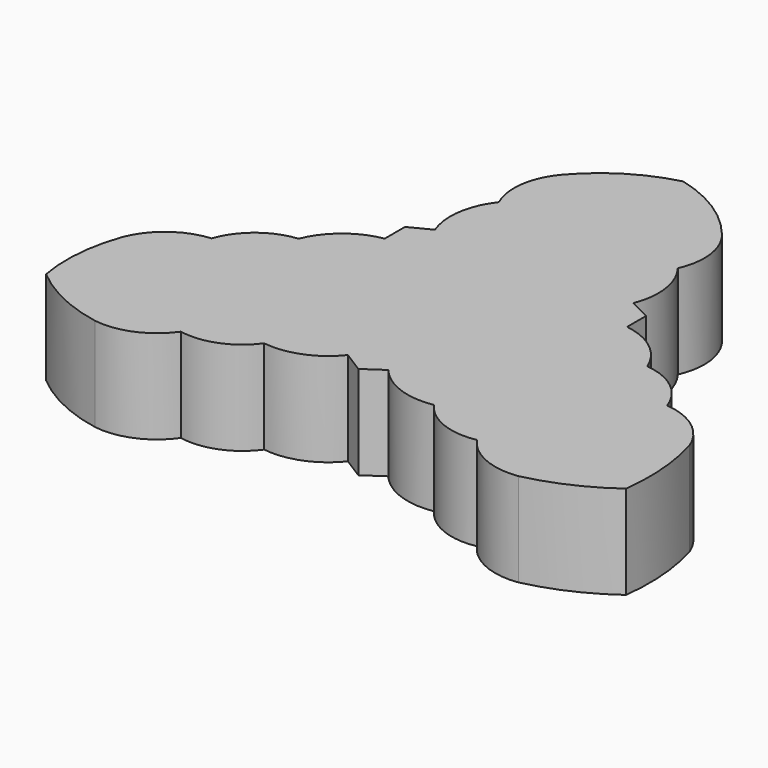
from build123d import *

# Parameters (mm, degrees)
F1_DEPTH = 9.525


# Not quite as in the source:
# - a length typed as a fraction of an inch, garbled in the dataset ("3 / 203.2 mm" for 3/8 in), is restored


with BuildPart() as f1:
    # F0 (on Top) → F1 (new body)
    with BuildSketch(Plane.XY):
        with BuildLine():
            ThreePointArc((0, 27.0671695471), (-4.5048536548, 25.1556778504), (-8.2258973271, 21.977417171))
            ThreePointArc((-8.2258973271, 21.977417171), (-9.7181261566, 18.698842434), (-9.2097157612, 15.1327075437))
            ThreePointArc((-9.2097157612, 15.1327075437), (-10.6205392688, 11.8246856933), (-10.2093555033, 8.2519613206))
            Line((-10.2093555033, 8.2519613206), (-12.369341217, 7.1464567445))
            Line((-12.369341217, 7.1464567445), (-12.369341217, 4.6386048198))
            Line((-12.369341217, 4.6386048198), (-12.369341217, 4.5682978211))
            ThreePointArc((-12.369341217, 4.5682978211), (-15.5930977879, 3.1185654947), (-17.7027139134, 0.2823972963))
            ThreePointArc((-17.7027139134, 0.2823972963), (-21.0452825194, -1.0603738309), (-23.1384971151, -3.9919692741))
            ThreePointArc((-23.1384971151, -3.9919692741), (-26.5647165348, -5.2934051439), (-28.80180468, -8.19653302))
            ThreePointArc((-28.80180468, -8.19653302), (-29.7673344436, -12.5572908836), (-29.5614041388, -17.0189104974))
            ThreePointArc((-29.5614041388, -17.0189104974), (-25.7783661022, -19.4669407743), (-21.4921734029, -20.8571857766))
            ThreePointArc((-21.4921734029, -20.8571857766), (-17.8594468391, -20.3713745504), (-15.0192606046, -18.054899429))
            ThreePointArc((-15.0192606046, -18.054899429), (-11.4338171794, -17.7079201351), (-8.5996589687, -15.484556372))
            ThreePointArc((-8.5996589687, -15.484556372), (-5.0294162563, -15.0523544446), (-2.1409380715, -12.9098966718))
            Line((-2.1409380715, -12.9098966718), (0, -14.2561570176))
            Line((0, -14.2561570176), (1.9696742658, -12.9098966718))
            ThreePointArc((1.9696742658, -12.9098966718), (4.9392756736, -15.0084468105), (8.560301624, -15.3410370587))
            ThreePointArc((8.560301624, -15.3410370587), (11.3944598347, -17.5644008218), (14.9799032599, -17.9113801157))
            ThreePointArc((14.9799032599, -17.9113801157), (17.8200894944, -20.2278552371), (21.4528160582, -20.7136664634))
            ThreePointArc((21.4528160582, -20.7136664634), (25.6558468929, -19.2922500665), (29.4813849032, -17.0447733253))
            ThreePointArc((29.4813849032, -17.0447733253), (29.5836204245, -12.511977875), (28.7624473353, -8.0530137067))
            ThreePointArc((28.7624473353, -8.0530137067), (26.5253591901, -5.1498858306), (23.0991397704, -3.8484499608))
            ThreePointArc((23.0991397704, -3.8484499608), (21.0059251747, -0.9168545176), (17.6633565687, 0.4259166096))
            ThreePointArc((17.6633565687, 0.4259166096), (15.4847616458, 3.3168082822), (12.1560195839, 4.739132713))
            Line((12.1560195839, 4.739132713), (12.1560195839, 7.1464567445))
            Line((12.1560195839, 7.1464567445), (9.9960338703, 8.2519613206))
            ThreePointArc((9.9960338703, 8.2519613206), (10.4072176357, 11.8246856933), (8.9963941282, 15.1327075437))
            ThreePointArc((8.9963941282, 15.1327075437), (9.5048045235, 18.698842434), (8.012575694, 21.977417171))
            ThreePointArc((8.012575694, 21.977417171), (4.4155385291, 25.1665589), (0, 27.0671695471))
        make_face()
    extrude(amount=F1_DEPTH)


solid = f1.part
